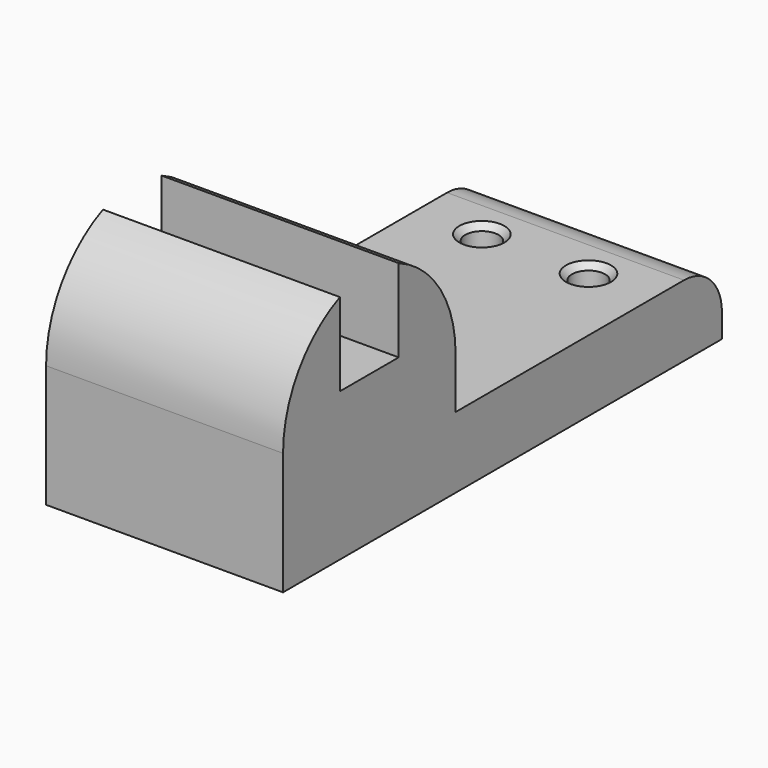
from build123d import *

# Parameters (mm, degrees)
F0_W        = 10
F0_H        = 28.1
F0_R        = 1.4
F1_DEPTH    = 6
F0_H_2      = 6
F2_DEPTH    = 19.5
F0_H_3      = 6.2
F0_R_2      = 2.1
F3_DEPTH    = 12.5
F4_DEPTH    = 19.5
F5_DEPTH    = 12.5
F6_DEPTH    = 6.5
F7_T1_DEPTH = 55.8257569496
F8_S5_R     = 1.4
F8_T6_DEPTH = 5
F9_R        = 4
F10_SIZE    = 0.5


# Not quite as in the source:
# - a fillet or chamfer that OpenCascade refuses, or shapes differently, is made with other operations: its cross-section is extruded or revolved along the edge and cut away or added


with BuildPart() as f1:
    # F0 (on Top) → F1 (new body)
    with BuildSketch(Plane.XY):
        with Locations((-5, -11.2607904853)):
            Rectangle(F0_W, F0_H)
        with Locations((-4.5, -4.4107904853)):
            Circle(F0_R, mode=Mode.SUBTRACT)
    extrude(amount=F1_DEPTH)

    # F0 (on Top) → F2 (join)
    with BuildSketch(Plane.XY):
        with Locations((-5, -28.3107904853)):
            Rectangle(F0_W, F0_H_2)
    extrude(amount=F2_DEPTH)

    # F0 (on Top) → F3 (join)
    with BuildSketch(Plane.XY):
        with Locations((-5, -34.4107904853)):
            Rectangle(F0_W, F0_H_3)
        with Locations((-4.5, -34.4107904853)):
            Circle(F0_R_2, mode=Mode.SUBTRACT)
    extrude(amount=F3_DEPTH)

    # F0 (on Top) → F4 (join)
    with BuildSketch(Plane.XY):
        with Locations((-5, -40.5107904853)):
            Rectangle(F0_W, F0_H_2)
    extrude(amount=F4_DEPTH)

    # F0 (on Top) → F5 (join)
    with BuildSketch(Plane.XY):
        with Locations((-4.5, -34.4107904853)):
            Circle(F0_R_2)
        with Locations((-4.5, -34.4107904853)):
            Circle(F0_R, mode=Mode.SUBTRACT)
    extrude(amount=F5_DEPTH)

    # F0 (on Top) → F6 (cut)
    with BuildSketch(Plane.XY):
        with Locations((-4.5, -34.4107904853)):
            Circle(F0_R_2)
        with Locations((-4.5, -34.4107904853)):
            Circle(F0_R, mode=Mode.SUBTRACT)
    extrude(amount=F6_DEPTH, mode=Mode.SUBTRACT)

    # F7: fillet of radius 10 on 2 edges, made by hand

    # F7_s2 → F7_t1 (cut)
    with BuildSketch(Plane.YZ.offset(-32.9128784748)):
        with BuildLine():
            ThreePointArc((-31.3107904853, 19.5), (-26.9441902199, 15.8120741851), (-25.3107904853, 10.3348486101))
            Line((-25.3107904853, 10.3348486101), (-25.3107904853, 19.5))
            Line((-25.3107904853, 19.5), (-31.3107904853, 19.5))
        make_face()
        with BuildLine():
            ThreePointArc((-43.5107904853, 10.3348486101), (-41.8773907506, 15.8120741851), (-37.5107904853, 19.5))
            Line((-37.5107904853, 19.5), (-43.5107904853, 19.5))
            Line((-43.5107904853, 19.5), (-43.5107904853, 10.3348486101))
        make_face()
    extrude(amount=F7_T1_DEPTH, mode=Mode.SUBTRACT)

    # F8: chamfer of 2 on 1 edges, made by hand


with BuildPart() as f8_tool2:
    # F8_s3 → F8_t4 (revolve)
    with BuildSketch(Plane.XZ.offset(34.4107904853)):
        Polygon((-2.4, 4.5), (-4.4, 6.5), (-2.4, 6.5), align=None)
    revolve(axis=Axis((-4.5, -34.4107904853, 6.5), (0, 0, 1)))

    # F8_s5 → F8_t6 (cut, symmetric)
    with BuildSketch(Plane.XY.offset(5.5)):
        with Locations((-4.5, -34.4107904853)):
            Circle(F8_S5_R)
    extrude(amount=F8_T6_DEPTH, both=True, mode=Mode.SUBTRACT)


with BuildPart() as f1_1:
    add(f1.part)

    # F8_t1: union F8_tool2
    add(f8_tool2.part)

    # F9
    f9_edges = [f1_1.edges().sort_by_distance(p)[0] for p in [
        (-5, 2.78921, 6),
    ]]
    fillet(f9_edges, radius=F9_R)

    # F10
    f10_edges = [f1_1.edges().sort_by_distance(p)[0] for p in [
        (-5.9, -4.41079, 6),
    ]]
    chamfer(f10_edges, length=F10_SIZE)

    # F11: F1 across plane


with BuildPart() as f1_2:
    add(f1_1.part)
    add(f1_1.part.mirror(Plane.YZ))


solid = f1_2.part
